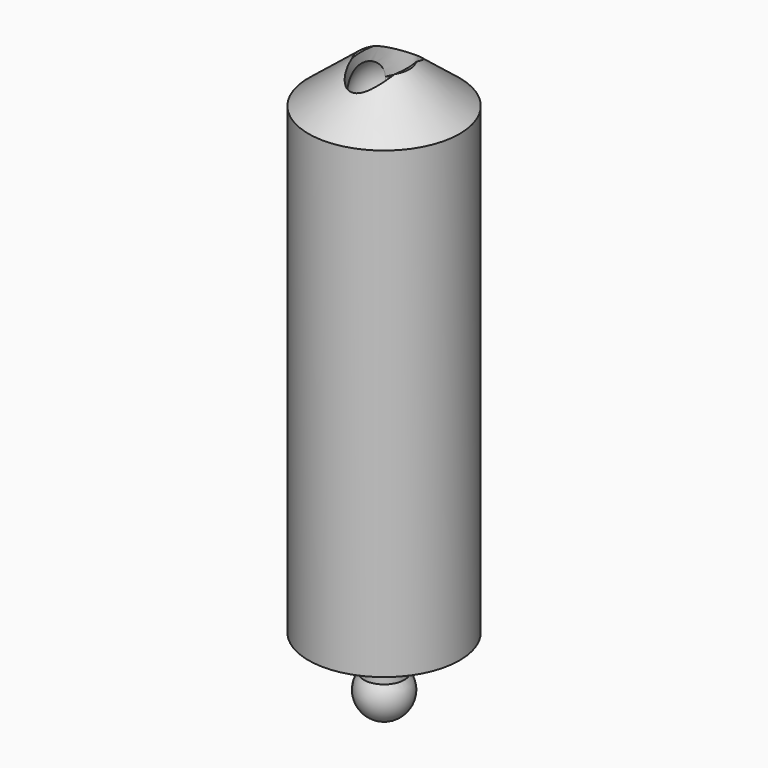
from build123d import *

# Parameters (mm, degrees)
F0_R     = 7.5
F1_DEPTH = 50
F2_R     = 2
F3_DEPTH = 5
F7_DEPTH = 3


# Not quite as in the source:
# - a fillet or chamfer that OpenCascade refuses, or shapes differently, is made with other operations: its cross-section is extruded or revolved along the edge and cut away or added


with BuildPart() as f1:
    # F0 (on Top) → F1 (new body)
    with BuildSketch(Plane.XY):
        Circle(F0_R)
    extrude(amount=F1_DEPTH)

    # F2 (on face) → F3 (join)
    with BuildSketch(Plane(origin=(0, 0, 0), x_dir=(1, 0, 0), z_dir=(0, 0, -1))):
        Circle(F2_R)
    extrude(amount=F3_DEPTH)

    # F4 (on face) → F5 (revolve)
    with BuildSketch(Plane(origin=(0, 0, -5), x_dir=(1, 0, 0), z_dir=(0, 0, -1))):
        with BuildLine():
            Line((0, 2), (0, 2.5))
            ThreePointArc((0, 2.5), (-2.5, 0), (0, -2.5))
            Line((0, -2.5), (0, -2))
            ThreePointArc((0, -2), (-2, 0), (0, 2))
        make_face()
    revolve(axis=Axis((0, 0, -5), (0, 1, 0)))

    # F6 (on face) → F7 (cut)
    with BuildSketch(Plane.XY.offset(50)):
        with BuildLine():
            add(Edge.make_bspline(
                [(0, 4), (-3.897114317, 4), (-1.9485571585, -2), (0, -8), (1.9485571585, -2), (3.897114317, 4), (0, 4)],
                knots=[0, 0, 0, 2.0943951024, 2.0943951024, 4.1887902048, 4.1887902048, 6.2831853072, 6.2831853072, 6.2831853072], degree=2, weights=[1, 0.5, 1, 0.5, 1, 0.5, 1]))
        make_face()
    extrude(amount=-F7_DEPTH, mode=Mode.SUBTRACT)

    # F8 (on face) → F9 (revolve, cut)
    with BuildSketch(Plane.XY.offset(47)):
        with BuildLine():
            ThreePointArc((1.8, -2.4), (2.683281573, -1.3416407865), (3, 0))
            ThreePointArc((3, 0), (2.683281573, 1.3416407865), (1.8, 2.4))
            add(Edge.make_bspline(
                [(1.8, -2.4), (1.8810311774, -2.2079260981), (1.9485571585, -2), (2.6913429511, 0.2871870789), (1.8, 2.4)],
                knots=[4.0484923357, 4.0484923357, 4.0484923357, 4.1887902048, 4.1887902048, 5.3448576064, 5.3448576064, 5.3448576064], degree=2, weights=[0.9375, 0.9665063509, 1, 0.7240092377, 0.7527020789]))
        make_face()
        with BuildLine():
            Line((0, -3), (0, 3))
            ThreePointArc((0, 3), (-0.9486832981, 2.8460498942), (-1.8, 2.4))
            add(Edge.make_bspline(
                [(-1.8, 2.4), (-2.6913429511, 0.2871870789), (-1.9485571585, -2), (-1.8810311774, -2.2079260981), (-1.8, -2.4)],
                knots=[0.9383277008, 0.9383277008, 0.9383277008, 2.0943951024, 2.0943951024, 2.2346929715, 2.2346929715, 2.2346929715], degree=2, weights=[0.7527020789, 0.7240092377, 1, 0.9665063509, 0.9375]))
            ThreePointArc((-1.8, -2.4), (-0.9486832981, -2.8460498942), (0, -3))
        make_face()
    revolve(axis=Axis((0, 0, 47), (0, -1, 0)), mode=Mode.SUBTRACT)

    # F10: chamfer of 5 x 4 on 1 edges, made by hand

    # F10_s1 → F10_t2 (revolve, cut)
    with BuildSketch(Plane.XZ):
        Polygon((7.5, 46), (2.5, 50), (7.5, 50), align=None)
    revolve(axis=Axis((0, 0, 50), (0, 0, 1)), mode=Mode.SUBTRACT)


solid = f1.part
